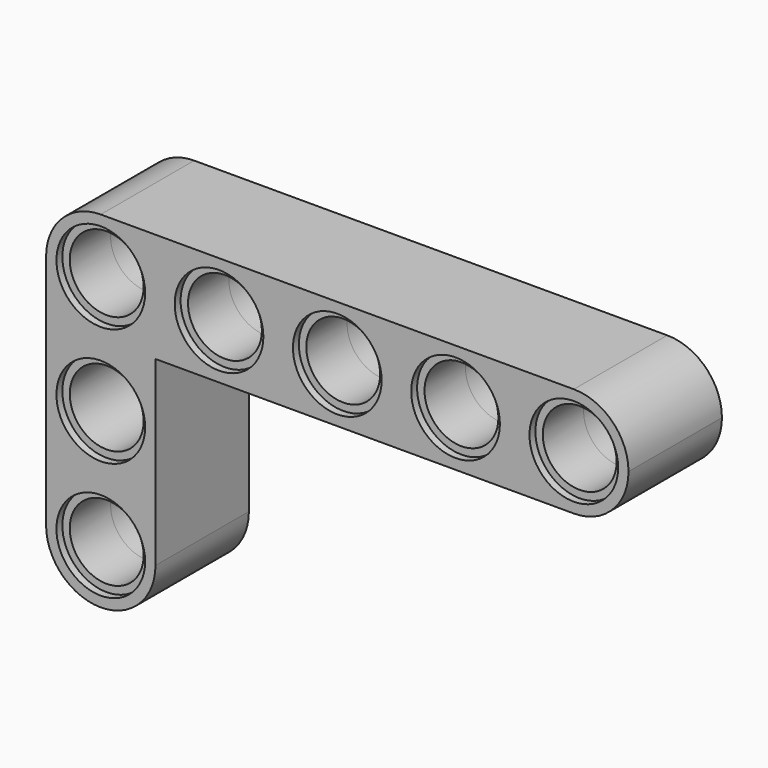
from build123d import *

# Parameters (mm, degrees)
F0_R     = 3
F1_DEPTH = 3.95
F0_R_2   = 2.499
F2_DEPTH = 3.45
F3_R     = 3.69999
F4_R     = 3.7


# Not quite as in the source:
# - a fillet or chamfer is up to 0.001 mm smaller than in the source, because OpenCascade refuses the exact size


with BuildPart() as f1:
    # F0 (on Front) → F1 (new body, symmetric)
    with BuildSketch(Plane.XZ):
        Polygon((19.7, 0), (-19.7, 0), (-19.7, -23.4), (-12.3, -23.4), (-12.3, -7.4), (19.7, -7.4), align=None)
        with Locations((-16, -19.7)):
            Circle(F0_R, mode=Mode.SUBTRACT)
        with Locations((-16, -11.7)):
            Circle(F0_R, mode=Mode.SUBTRACT)
        with Locations((-16, -3.7)):
            Circle(F0_R, mode=Mode.SUBTRACT)
        with Locations((-8, -3.7)):
            Circle(F0_R, mode=Mode.SUBTRACT)
        with Locations((0, -3.7)):
            Circle(F0_R, mode=Mode.SUBTRACT)
        with Locations((8, -3.7)):
            Circle(F0_R, mode=Mode.SUBTRACT)
        with Locations((16, -3.7)):
            Circle(F0_R, mode=Mode.SUBTRACT)
    extrude(amount=F1_DEPTH, both=True)

    # F0 (on Front) → F2 (join, symmetric)
    with BuildSketch(Plane.XZ):
        with Locations((16, -3.7)):
            Circle(F0_R)
        with Locations((16, -3.7)):
            Circle(F0_R_2, mode=Mode.SUBTRACT)
        with Locations((8, -3.7)):
            Circle(F0_R)
        with Locations((8, -3.7)):
            Circle(F0_R_2, mode=Mode.SUBTRACT)
        with Locations((0, -3.7)):
            Circle(F0_R)
        with Locations((0, -3.7)):
            Circle(F0_R_2, mode=Mode.SUBTRACT)
        with Locations((-8, -3.7)):
            Circle(F0_R)
        with Locations((-8, -3.7)):
            Circle(F0_R_2, mode=Mode.SUBTRACT)
        with Locations((-16, -3.7)):
            Circle(F0_R)
        with Locations((-16, -3.7)):
            Circle(F0_R_2, mode=Mode.SUBTRACT)
        with Locations((-16, -19.7)):
            Circle(F0_R)
        with Locations((-16, -19.7)):
            Circle(F0_R_2, mode=Mode.SUBTRACT)
        with Locations((-16, -11.7)):
            Circle(F0_R)
        with Locations((-16, -11.7)):
            Circle(F0_R_2, mode=Mode.SUBTRACT)
    extrude(amount=F2_DEPTH, both=True)

    # F3 (radius 3.7 in the source; OpenCascade refuses exactly that, so slightly less here)
    f3_edges = [f1.edges().sort_by_distance(p)[0] for p in [
        (19.7, 0, 0),
        (19.7, 0, -7.4),
        (-12.3, 0, -23.4),
        (-19.7, 0, -23.4),
    ]]
    fillet(f3_edges, radius=F3_R)

    # F4
    f4_edges = [f1.edges().sort_by_distance(p)[0] for p in [
        (-19.7, 0, 0),
    ]]
    fillet(f4_edges, radius=F4_R)


solid = f1.part
